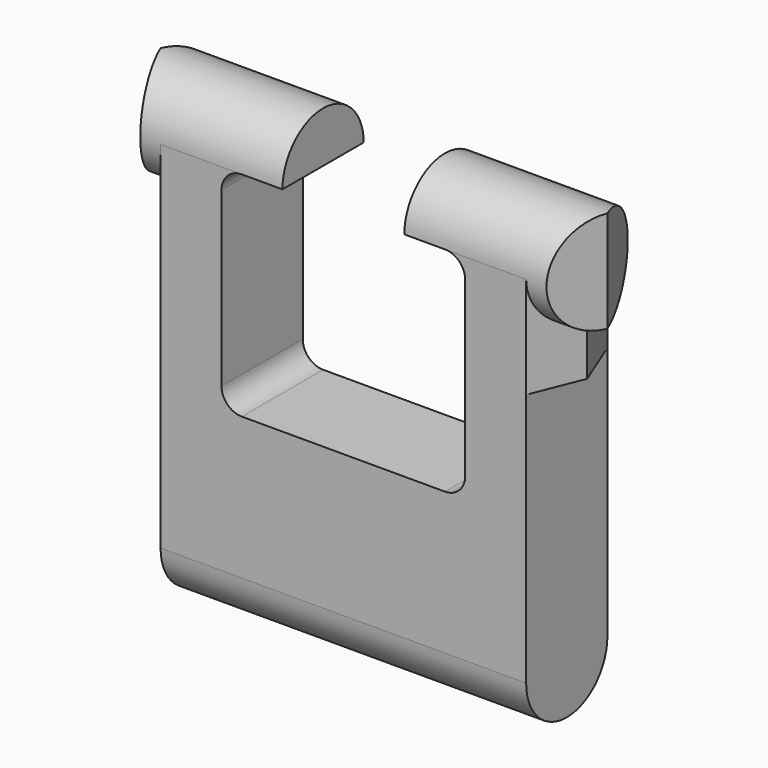
from build123d import *

# Parameters (mm, degrees)
F2_DEPTH    = 2.5
F3_DEPTH    = 10
F4_DEPTH    = 3
F5_DEPTH    = 6
F6_T1_DEPTH = 5
F8_DEPTH    = 14
F9_DEPTH    = 9
F10_DEPTH   = 1
F11_DEPTH   = 16.5
F13_DEPTH   = 6
F14_R       = 2.49999


# Not quite as in the source:
# - a fillet or chamfer that OpenCascade refuses, or shapes differently, is made with other operations: its cross-section is extruded or revolved along the edge and cut away or added
# - a fillet or chamfer is up to 0.001 mm smaller than in the source, because OpenCascade refuses the exact size


with BuildPart() as f2:
    # F0 (on Front) → F2 (new body, symmetric)
    with BuildSketch(Plane.XZ):
        Polygon((0, 3.5), (0, 0), (9, 0), (9, 14), (6, 14), (6, 3.5), align=None)
    extrude(amount=F2_DEPTH, both=True)

    # F1 (on Right) → F3 (join)
    with BuildSketch(Plane.YZ):
        with BuildLine():
            Line((-2.5, 14), (2.5, 14))
            ThreePointArc((2.5, 14), (0, 16.5), (-2.5, 14))
        make_face()
        with BuildLine():
            ThreePointArc((-2.5, 14), (0, 11.5), (2.5, 14))
            Line((2.5, 14), (-2.5, 14))
        make_face()
    extrude(amount=F3_DEPTH)

    # F1 (on Right) → F4 (cut)
    with BuildSketch(Plane.YZ):
        with BuildLine():
            Line((-2.5, 14), (2.5, 14))
            ThreePointArc((2.5, 14), (0, 16.5), (-2.5, 14))
        make_face()
        with BuildLine():
            ThreePointArc((-2.5, 14), (0, 11.5), (2.5, 14))
            Line((2.5, 14), (-2.5, 14))
        make_face()
    extrude(amount=F4_DEPTH, mode=Mode.SUBTRACT)

    # F1 (on Right) → F5 (cut)
    with BuildSketch(Plane.YZ):
        with BuildLine():
            ThreePointArc((-2.5, 14), (0, 11.5), (2.5, 14))
            Line((2.5, 14), (-2.5, 14))
        make_face()
    extrude(amount=F5_DEPTH, mode=Mode.SUBTRACT)

    # F6: fillet of radius 1 on 2 edges, made by hand

    # F6_s2 → F6_t1 (join)
    with BuildSketch(Plane.XZ.offset(-2.5)):
        with BuildLine():
            ThreePointArc((6, 13), (5.7071067812, 13.7071067812), (5, 14))
            Line((5, 14), (6, 14))
            Line((6, 14), (6, 13))
        make_face()
        with BuildLine():
            ThreePointArc((5, 3.5), (5.7071067812, 3.7928932188), (6, 4.5))
            Line((6, 4.5), (6, 3.5))
            Line((6, 3.5), (5, 3.5))
        make_face()
    extrude(amount=F6_T1_DEPTH)

    # F7 (on Top) → F8 (join)
    with BuildSketch(Plane.XY):
        Polygon((9, 2.5), (9, -2.5), (10, 0), align=None)
    extrude(amount=F8_DEPTH)

    # F7 (on Top) → F9 (cut)
    with BuildSketch(Plane.XY):
        Polygon((9, 2.5), (9, -2.5), (10, 0), align=None)
    extrude(amount=F9_DEPTH, mode=Mode.SUBTRACT)

    # F10 (add): a face of the model
    f10_faces = [f2.faces().sort_by_distance(p)[0] for p in [
        (10, -1.717766953, 12.282233047),
    ]]
    extrude(f10_faces, amount=F10_DEPTH)

    # F7 (on Top) → F11 (cut)
    with BuildSketch(Plane.XY):
        Polygon((11, 0), (10, -2.5), (11.5, -2.5), (11.5, 2.5), (10, 2.5), align=None)
    extrude(amount=F11_DEPTH, mode=Mode.SUBTRACT)

    # F12: F2 across face


with BuildPart() as f2_1:
    add(f2.part)
    add(f2.part.mirror(Plane(origin=(0, 0, 1.75), x_dir=(0, -1, 0), z_dir=(-1, 0, 0))))

    # F13 (add): a face of the model
    f13_faces = [f2_1.faces().sort_by_distance(p)[0] for p in [
        (0, 0, 0),
    ]]
    extrude(f13_faces, amount=F13_DEPTH)

    # F14 (radius 2.5 in the source; OpenCascade refuses exactly that, so slightly less here)
    f14_edges = [f2_1.edges().sort_by_distance(p)[0] for p in [
        (0, -2.5, -6),
        (0, 2.5, -6),
    ]]
    fillet(f14_edges, radius=F14_R)


solid = f2_1.part
